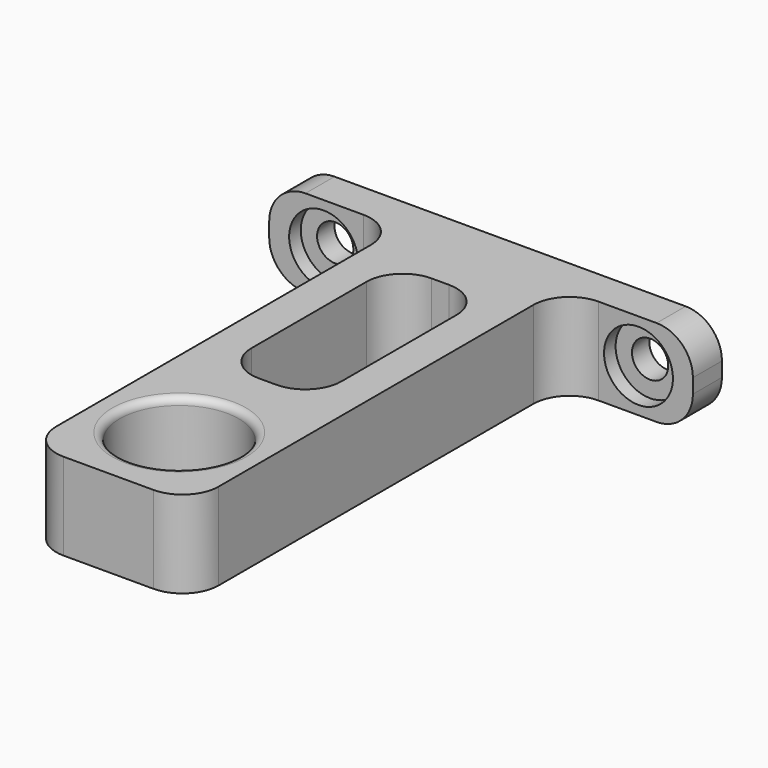
from build123d import *

# Parameters (mm, degrees)
F0_W     = 12.4
F0_H     = 29.8
F1_DEPTH = 12
F2_W     = 58.4
F2_H     = 12
F2_R     = 2.5
F3_DEPTH = 5
F4_R     = 5
F5_R     = 5
F6_R     = 5
F7_R     = 4.75
F8_DEPTH = 2
F9_R     = 1
F10_R    = 5


# Not quite as in the source:
# - a feature names something its author has since deleted; it is built from what else it names


with BuildPart() as f1:
    # F0 (on Top) → F1 (new body)
    with BuildSketch(Plane.XY):
        with BuildLine():
            ThreePointArc((-8.2, 0), (0, 8.2), (8.2, 0))
            Line((8.2, 0), (11.2, 0))
            Line((11.2, 0), (11.2, 52))
            Line((11.2, 52), (0, 52))
            Line((0, 52), (-11.2, 52))
            Line((-11.2, 52), (-11.2, 0))
            Line((-11.2, 0), (-8.2, 0))
        make_face()
        with Locations((0, 30.1)):
            Rectangle(F0_W, F0_H, mode=Mode.SUBTRACT)
        with BuildLine():
            Line((11.2, 0), (8.2, 0))
            ThreePointArc((8.2, 0), (0, -8.2), (-8.2, 0))
            Line((-8.2, 0), (-11.2, 0))
            Line((-11.2, 0), (-11.2, -12.2))
            Line((-11.2, -12.2), (0, -12.2))
            Line((0, -12.2), (11.2, -12.2))
            Line((11.2, -12.2), (11.2, 0))
        make_face()
        with BuildLine():
            Line((11.2, 0), (8.2, 0))
            ThreePointArc((8.2, 0), (0, -8.2), (-8.2, 0))
            Line((-8.2, 0), (-11.2, 0))
            Line((-11.2, 0), (-11.2, -12.2))
            Line((-11.2, -12.2), (0, -12.2))
            Line((0, -12.2), (11.2, -12.2))
            Line((11.2, -12.2), (11.2, 0))
        make_face()
    extrude(amount=F1_DEPTH)

    # F2 (on face) → F3 (join)
    with BuildSketch(Plane(origin=(0, 52, 0), x_dir=(-1, 0, 0), z_dir=(0, 1, 0))):
        with Locations((0, 6)):
            Rectangle(F2_W, F2_H)
        with Locations((-21.7, 6)):
            Circle(F2_R, mode=Mode.SUBTRACT)
        with Locations((21.7, 6)):
            Circle(F2_R, mode=Mode.SUBTRACT)
    extrude(amount=F3_DEPTH)

    # F4
    f4_edges = [f1.edges().sort_by_distance(p)[0] for p in [
        (-11.2, -12.2, 6),
        (11.2, -12.2, 6),
    ]]
    fillet(f4_edges, radius=F4_R)

    # F5
    f5_edges = [f1.edges().sort_by_distance(p)[0] for p in [
        (11.2, 52, 6),
        (-11.2, 52, 6),
    ]]
    fillet(f5_edges, radius=F5_R)

    # F6
    f6_edges = [f1.edges().sort_by_distance(p)[0] for p in [
        (-29.2, 54.5, 12),
        (-29.2, 54.5, 0),
        (29.2, 54.5, 0),
        (29.2, 54.5, 12),
    ]]
    fillet(f6_edges, radius=F6_R)

    # F7 (on face) → F8 (cut)
    with BuildSketch(Plane.XZ.offset(-52)):
        with Locations((21.7, 6)):
            Circle(F7_R)
        with Locations((-21.7, 6)):
            Circle(F7_R)
    extrude(amount=-F8_DEPTH, mode=Mode.SUBTRACT)

    # F9
    f9_edges = [f1.edges().sort_by_distance(p)[0] for p in [
        (8.2, 0, 12),
    ]]
    fillet(f9_edges, radius=F9_R)

    # F10
    f10_edges = [f1.edges().sort_by_distance(p)[0] for p in [
        (-6.2, 45, 6),
        (6.2, 45, 6),
        (-6.2, 15.2, 6),
        (6.2, 15.2, 6),
    ]]
    fillet(f10_edges, radius=F10_R)


solid = f1.part
